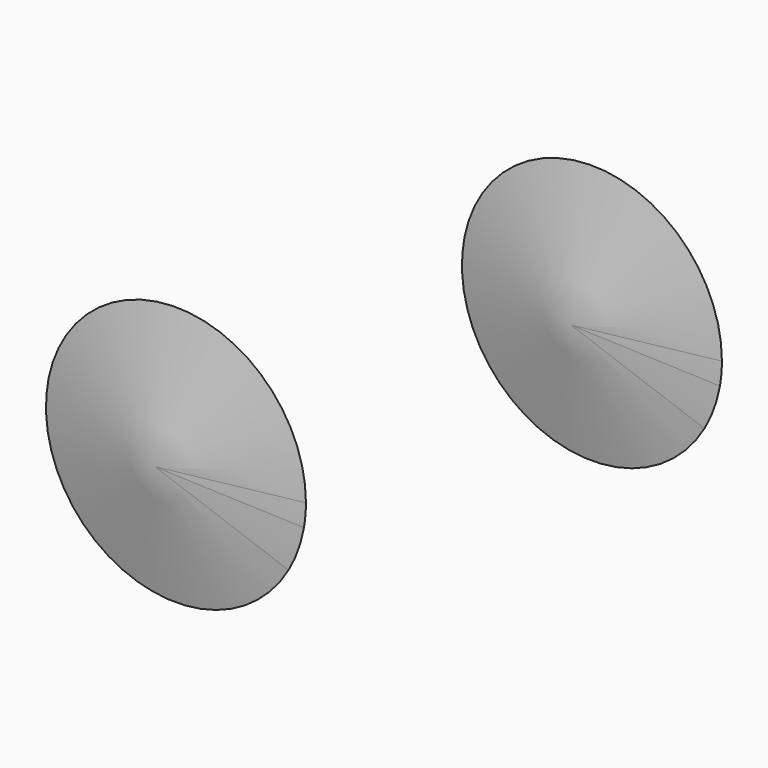
from build123d import *
from build123d import SkipClean  # not in build123d's __all__

# Parameters (mm, degrees)
F0_R     = 63.5
F1_DEPTH = 25.4
F4_ANGLE = 350
F6_ANGLE = 30


with BuildPart() as f1:
    # F0 (on Front) → F1 (new body)
    with BuildSketch(Plane.XZ):
        Circle(F0_R)
    extrude(amount=F1_DEPTH)

    # F2 (on Top) → F4 (revolve, cut)
    with BuildSketch(Plane.XY):
        Polygon((63.5, -25.4), (63.5, -12.7), (0, -25.4), align=None)
        Polygon((63.5, -12.7), (63.5, 0), (0, 0), align=None)
    revolve(axis=Axis((0, 21.4261654764, 0), (0, -1, 0)), revolution_arc=F4_ANGLE, mode=Mode.SUBTRACT)

    # F5 (on face) → F6 (revolve, cut)
    with BuildSketch(Plane.XY):
        Polygon((63.5, 0), (0, 0), (63.5, -12.7), align=None)
        Polygon((63.5, -25.4), (63.5, -12.7), (0, -25.4), align=None)
    with SkipClean():  # cleaning this boolean's faces spoils the solid; the shape is the same uncleaned
        revolve(axis=Axis((0, 21.4261654764, 0), (0, 1, 0)), revolution_arc=F6_ANGLE, mode=Mode.SUBTRACT)


with BuildPart() as f7_1:
    # F7: copy of F1
    add(f1.part, clean=False)


with BuildPart() as f7_1_1:
    # F8: moved
    add(f7_1.part.moved(Location((203.2, 0, 127))), clean=False)


solid = Compound([f1.part, f7_1_1.part])
